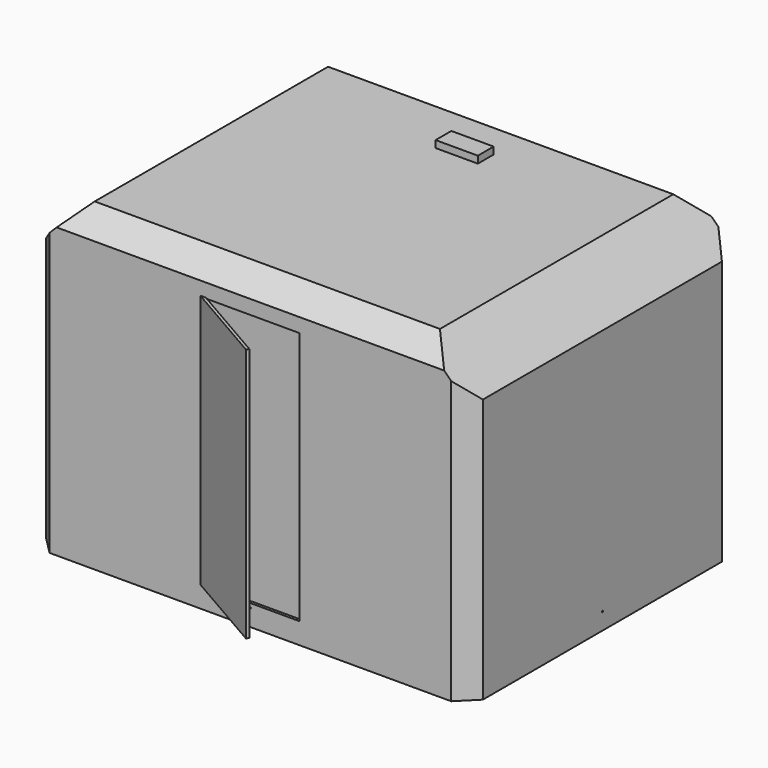
from build123d import *

# Parameters (mm, degrees)
F0_W           = 3100
F0_H           = 2200
F1_DEPTH       = 2370
F2_SIZE        = 325
F3_SIZE        = 325
F4_SIZE        = 125
F5_SIZE        = 125
F6_SIZE        = 125
F7_SIZE        = 125
F8_W           = 1500
F8_H           = 1300
F9_DEPTH       = 120
F10_W          = 400
F10_H          = 200
F10_R          = 7.5
F11_DEPTH      = 1
F12_R          = 5
F13_DEPTH      = 1
F14_DEPTH      = 800.001
F14_DEPTH_BACK = 2300.001
F15_R          = 5
F16_DEPTH      = 535.001
F16_DEPTH_BACK = 1835.001
F17_SIZE       = 150
F18_SIZE       = 150
F19_W          = 1700
F19_H          = 1500
F19_W_2        = 1500
F19_H_2        = 1300
F20_DEPTH      = 10
F21_W          = 700
F21_H          = 1800
F22_DEPTH      = 20
F23_W          = 300
F23_H          = 140
F24_DEPTH      = 50
F26_DEPTH      = 1805


# Not quite as in the source:
# - a feature of the source that left no trace in its solid (it failed there, or was rolled back) is left out


with BuildPart() as f1:
    # F0 (on Front) → F1 (new body)
    with BuildSketch(Plane.XZ):
        Rectangle(F0_W, F0_H)
    extrude(amount=F1_DEPTH)

    # F2
    f2_edges = [f1.edges().sort_by_distance(p)[0] for p in [
        (-1550, -1185, 1100),
    ]]
    chamfer(f2_edges, length=F2_SIZE)

    # F3
    f3_edges = [f1.edges().sort_by_distance(p)[0] for p in [
        (1550, -1185, 1100),
    ]]
    chamfer(f3_edges, length=F3_SIZE)

    # F4
    f4_edges = [f1.edges().sort_by_distance(p)[0] for p in [
        (1550, -2370, -162.5),
    ]]
    chamfer(f4_edges, length=F4_SIZE)

    # F5
    f5_edges = [f1.edges().sort_by_distance(p)[0] for p in [
        (-1550, -2370, -162.5),
    ]]
    chamfer(f5_edges, length=F5_SIZE)

    # F6
    f6_edges = [f1.edges().sort_by_distance(p)[0] for p in [
        (-1550, 0, -162.5),
    ]]
    chamfer(f6_edges, length=F6_SIZE)

    # F7
    f7_edges = [f1.edges().sort_by_distance(p)[0] for p in [
        (1550, 0, -162.5),
    ]]
    chamfer(f7_edges, length=F7_SIZE)

    # F8 (on face) → F9 (cut)
    with BuildSketch(Plane(origin=(0, 0, -1100), x_dir=(1, 0, 0), z_dir=(0, 0, -1))):
        with Locations((0, 1185)):
            Rectangle(F8_W, F8_H)
    extrude(amount=-F9_DEPTH, mode=Mode.SUBTRACT)

    # F10 (on face) → F11 (cut)
    with BuildSketch(Plane(origin=(0, 0, -980), x_dir=(1, 0, 0), z_dir=(0, 0, -1))):
        with Locations((0, 1714)):
            Rectangle(F10_W, F10_H)
        with Locations((0, 1794)):
            Circle(F10_R, mode=Mode.SUBTRACT)
        Polygon((601.4287087912, 1118.7050807569), (428.2236280343, 1218.7050807569), (228.2236280343, 872.2949192431), (401.4287087912, 772.2949192431), align=None)
        with Locations((484.1082007155, 955.5)):
            Circle(F10_R, mode=Mode.SUBTRACT)
        Polygon((-228.2236280343, 872.2949192431), (-428.2236280343, 1218.7050807569), (-601.4287087912, 1118.7050807569), (-401.4287087912, 772.2949192431), align=None)
        with Locations((-484.1082007155, 955.5)):
            Circle(F10_R, mode=Mode.SUBTRACT)
        with Locations((0, 1235)):
            Circle(F10_R)
    extrude(amount=-F11_DEPTH, mode=Mode.SUBTRACT)

    # F12 (on face) → F13 (cut)
    with BuildSketch(Plane.YZ.offset(-750)):
        with Locations((-1185, -980)):
            Circle(F12_R)
    extrude(amount=F13_DEPTH, mode=Mode.SUBTRACT)

    # F12 (on face) → F14 (cut, two sides)
    with BuildSketch(Plane.YZ.offset(-750)) as f14_sk:
        with Locations((-1185, -980)):
            Circle(F12_R)
    extrude(amount=-F14_DEPTH, mode=Mode.SUBTRACT)
    extrude(f14_sk.sketch, amount=F14_DEPTH_BACK, mode=Mode.SUBTRACT)

    # F15 (on face) → F16 (cut, two sides)
    with BuildSketch(Plane.XZ.offset(535)) as f16_sk:
        with Locations((0, -980)):
            Circle(F15_R)
    extrude(amount=-F16_DEPTH, mode=Mode.SUBTRACT)
    extrude(f16_sk.sketch, amount=F16_DEPTH_BACK, mode=Mode.SUBTRACT)

    # F17
    f17_edges = [f1.edges().sort_by_distance(p)[0] for p in [
        (0, 0, 1100),
    ]]
    chamfer(f17_edges, length=F17_SIZE)

    # F18
    f18_edges = [f1.edges().sort_by_distance(p)[0] for p in [
        (0, -2370, 1100),
    ]]
    chamfer(f18_edges, length=F18_SIZE)

    # F19 (on face) → F20 (join)
    with BuildSketch(Plane(origin=(0, 0, -1100), x_dir=(1, 0, 0), z_dir=(0, 0, -1))):
        with Locations((0, 1185)):
            Rectangle(F19_W, F19_H)
        with Locations((0, 1185)):
            Rectangle(F19_W_2, F19_H_2, mode=Mode.SUBTRACT)
    extrude(amount=F20_DEPTH)

    # F21 (on face) → F22 (cut)
    with BuildSketch(Plane.XZ.offset(2370)):
        with Locations((0, -50)):
            Rectangle(F21_W, F21_H)
    extrude(amount=-F22_DEPTH, mode=Mode.SUBTRACT)

    # F23 (on face) → F24 (join)
    with BuildSketch(Plane.XY.offset(1100)):
        with Locations((0, -470)):
            Rectangle(F23_W, F23_H)
    extrude(amount=F24_DEPTH)

    # F25 (on face) → F26 (join)
    with BuildSketch(Plane.XY.offset(-950)):
        Polygon((-350, -2350), (-360, -2367.3205080757), (246.2177826491, -2717.3205080757), (256.2177826491, -2700), align=None)
    extrude(amount=F26_DEPTH)


solid = f1.part
